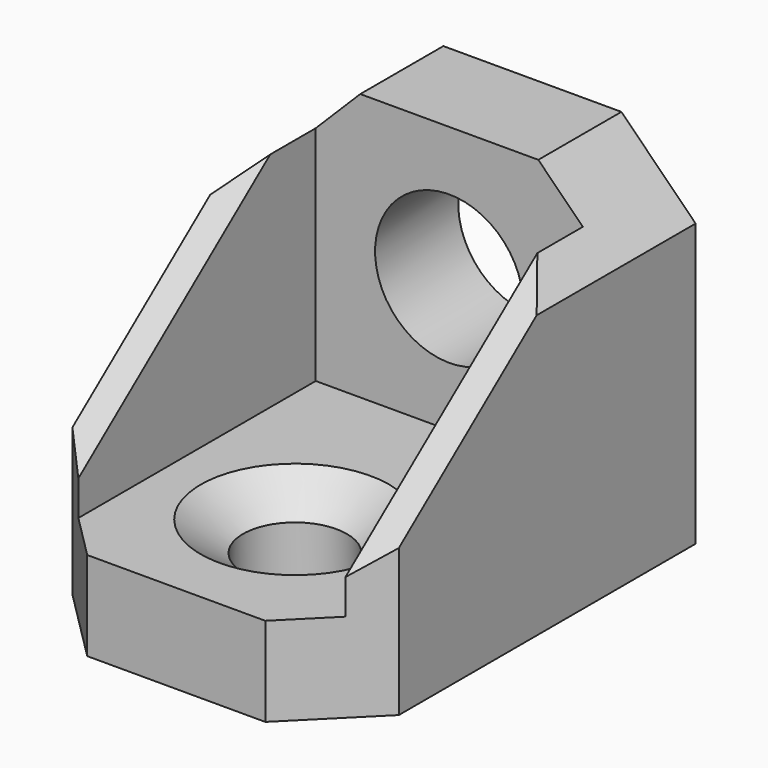
from build123d import *

# Parameters (mm, degrees)
F0_W        = 2
F0_H        = 23
F0_W_2      = 18
F0_R        = 3.5
F1_DEPTH    = 6
F2_DEPTH    = 18
F3_R        = 5
F4_DEPTH    = 25
F5_SIZE2    = 23
F5_SIZE     = 18
F6_T1_DEPTH = 31.7168298797
F6_T3_DEPTH = 32.7168298797
F7_SIZE2    = 2.8562960135
F7_SIZE     = 2


# Not quite as in the source:
# - a fillet or chamfer that OpenCascade refuses, or shapes differently, is made with other operations: its cross-section is extruded or revolved along the edge and cut away or added


with BuildPart() as f1:
    # F0 (on Top) → F1 (new body)
    with BuildSketch(Plane.XY):
        with Locations((-10, -3.5)):
            Rectangle(F0_W, F0_H)
        with Locations((0, -3.5)):
            Rectangle(F0_W_2, F0_H)
        with Locations((0, -5)):
            Circle(F0_R, mode=Mode.SUBTRACT)
        with Locations((10, -3.5)):
            Rectangle(F0_W, F0_H)
        Polygon((9, 8), (11, 8), (11, 15), (-11, 15), (-11, 8), (-9, 8), align=None)
    extrude(amount=-F1_DEPTH)

    # F0 (on Top) → F2 (join)
    with BuildSketch(Plane.XY):
        Polygon((9, 8), (11, 8), (11, 15), (-11, 15), (-11, 8), (-9, 8), align=None)
        with Locations((-10, -3.5)):
            Rectangle(F0_W, F0_H)
        with Locations((10, -3.5)):
            Rectangle(F0_W, F0_H)
    extrude(amount=F2_DEPTH)

    # F3 (on face) → F4 (cut)
    with BuildSketch(Plane.XZ.offset(-8)):
        with Locations((0, 9)):
            Circle(F3_R)
    extrude(amount=-F4_DEPTH, mode=Mode.SUBTRACT)

    # F5
    f5_edges = [f1.edges().sort_by_distance(p)[0] for p in [
        (-10, -15, 18),
        (10, -15, 18),
    ]]
    f5_side = f1.faces().sort_by_distance((0, -15, -5.674424))[0]
    chamfer(f5_edges, length=F5_SIZE, length2=F5_SIZE2, reference=f5_side)

    # F6: chamfer of 5 on 4 edges, made by hand

    # F6_s2 → F6_t1 (cut)
    with BuildSketch(Plane.XY.offset(-18.8584149398)):
        Polygon((6, -15), (11, -10), (11, -15), align=None)
        Polygon((-6, -15), (-11, -10), (-11, -15), align=None)
    extrude(amount=F6_T1_DEPTH, mode=Mode.SUBTRACT)

    # F6_s4 → F6_t3 (cut)
    with BuildSketch(Plane.XZ.offset(-27.8584149398)):
        Polygon((11, 13), (6, 18), (11, 18), align=None)
        Polygon((-11, 13), (-6, 18), (-11, 18), align=None)
    extrude(amount=F6_T3_DEPTH, mode=Mode.SUBTRACT)

    # F7
    f7_edges = [f1.edges().sort_by_distance(p)[0] for p in [
        (-3.5, -5, 0),
    ]]
    f7_side = f1.faces().sort_by_distance((-3.5, -5, -3))[0]
    chamfer(f7_edges, length=F7_SIZE, length2=F7_SIZE2, reference=f7_side)


solid = f1.part
